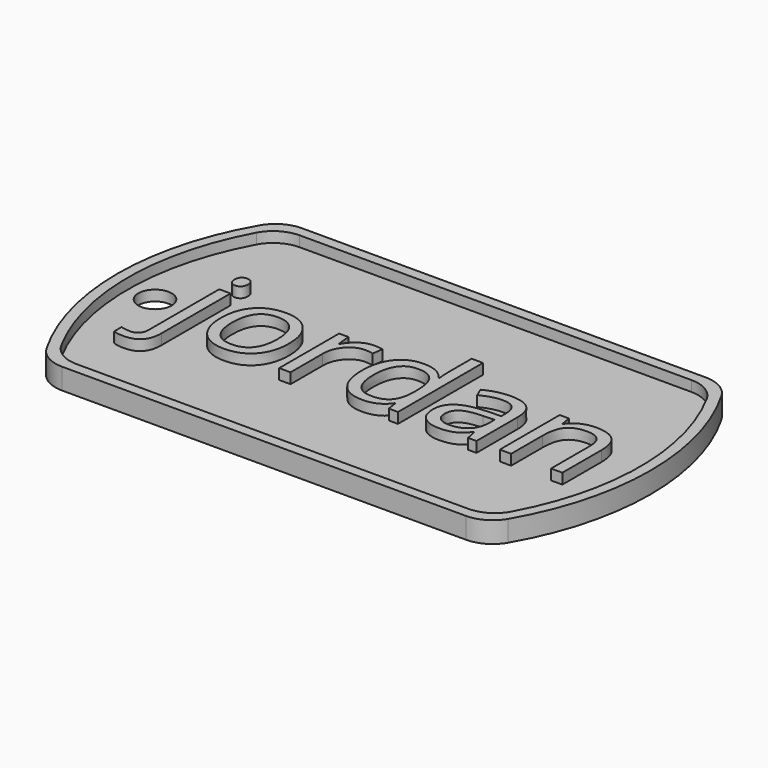
from build123d import *

# Parameters (mm, degrees)
F1_DEPTH     = 1
F3_DEPTH     = 1
F4_R         = 1.5875
F5_DEPTH     = 1
F6_TEXT_SIZE = 13.3282453236
F7_DEPTH     = 1


# Not quite as in the source:
# - Text() gives the source's letters only with a copy of the font that has no kerning and outlines rounded to 1/6400 em; it was checked with that copy


with BuildPart() as f1:
    # F0 (on Top) → F1 (new body)
    with BuildSketch(Plane.XY):
        with BuildLine():
            ThreePointArc((-19.2474145991, 14.2875), (-20.8349145991, 13.862130657), (-21.9970452561, 12.7))
            ThreePointArc((-21.9970452561, 12.7), (-25.4, 0), (-21.9970452561, -12.7))
            ThreePointArc((-21.9970452561, -12.7), (-20.8349145991, -13.862130657), (-19.2474145991, -14.2875))
            Line((-19.2474145991, -14.2875), (19.2474145991, -14.2875))
            ThreePointArc((19.2474145991, -14.2875), (20.8349145991, -13.862130657), (21.9970452561, -12.7))
            ThreePointArc((21.9970452561, -12.7), (25.4, 0), (21.9970452561, 12.7))
            ThreePointArc((21.9970452561, 12.7), (20.8349145991, 13.862130657), (19.2474145991, 14.2875))
            Line((19.2474145991, 14.2875), (-19.2474145991, 14.2875))
        make_face()
    extrude(amount=F1_DEPTH)

    # F2 (on face) → F3 (join)
    with BuildSketch(Plane.XY.offset(1)):
        with BuildLine():
            Line((19.2474145991, 14.2875), (-19.2474145991, 14.2875))
            ThreePointArc((-19.2474145991, 14.2875), (-20.8349145991, 13.862130657), (-21.9970452561, 12.7))
            ThreePointArc((-21.9970452561, 12.7), (-25.4, 0), (-21.9970452561, -12.7))
            ThreePointArc((-21.9970452561, -12.7), (-20.8349145991, -13.862130657), (-19.2474145991, -14.2875))
            Line((-19.2474145991, -14.2875), (19.2474145991, -14.2875))
            ThreePointArc((19.2474145991, -14.2875), (20.8349145991, -13.862130657), (21.9970452561, -12.7))
            ThreePointArc((21.9970452561, -12.7), (25.4, 0), (21.9970452561, 12.7))
            ThreePointArc((21.9970452561, 12.7), (20.8349145991, 13.862130657), (19.2474145991, 14.2875))
        make_face()
        with BuildLine():
            ThreePointArc((-21.4526124879, 11.6252061249), (-20.2856017842, 12.8404540819), (-18.6611352482, 13.2875))
            Line((-18.6611352482, 13.2875), (18.6611352482, 13.2875))
            ThreePointArc((18.6611352482, 13.2875), (20.2856017842, 12.8404540819), (21.4526124879, 11.6252061249))
            ThreePointArc((21.4526124879, 11.6252061249), (24.4, 0), (21.4526124879, -11.6252061249))
            ThreePointArc((21.4526124879, -11.6252061249), (20.2856017842, -12.8404540819), (18.6611352482, -13.2875))
            Line((18.6611352482, -13.2875), (-18.6611352482, -13.2875))
            ThreePointArc((-18.6611352482, -13.2875), (-20.2856017842, -12.8404540819), (-21.4526124879, -11.6252061249))
            ThreePointArc((-21.4526124879, -11.6252061249), (-24.4, 0), (-21.4526124879, 11.6252061249))
        make_face(mode=Mode.SUBTRACT)
    extrude(amount=F3_DEPTH)

    # F4 (on face) → F5 (cut)
    with BuildSketch(Plane.XY.offset(1)):
        with Locations((-21.821282804, 0)):
            Circle(F4_R)
    extrude(amount=-F5_DEPTH, mode=Mode.SUBTRACT)

    # F6 (on face) → F7 (join)
    with BuildSketch(Plane.XY.offset(1)):
        with Locations((-19.0582049545, -4.3709441088)):
            Text('jordan', F6_TEXT_SIZE, font='Open Sans', text_align=(TextAlign.LEFT, TextAlign.BOTTOM))
    extrude(amount=F7_DEPTH)


solid = f1.part
